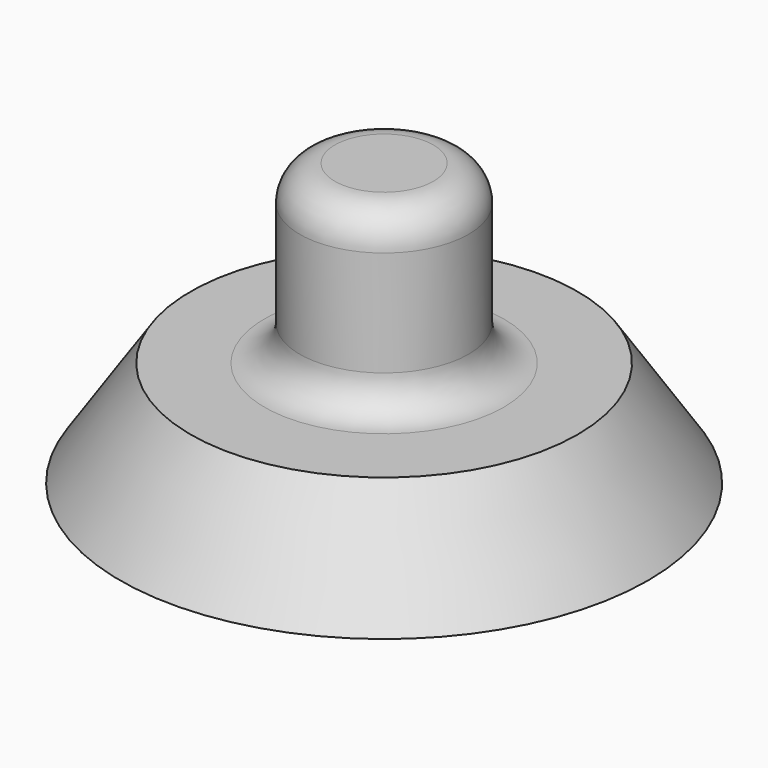
from build123d import *

# Parameters (mm, degrees)
F0_R     = 7.5
F1_DEPTH = 3
F2_SIZE2 = 2.99999
F2_SIZE  = 1.99999
F3_R     = 2.4
F4_DEPTH = 5
F5_R     = 1


# Not quite as in the source:
# - a fillet or chamfer is up to 0.001 mm smaller than in the source, because OpenCascade refuses the exact size


with BuildPart() as f1:
    # F0 (on Top) → F1 (new body)
    with BuildSketch(Plane.XY):
        Circle(F0_R)
    extrude(amount=F1_DEPTH)

    # F2 (size 2 and 3 in the source; OpenCascade refuses exactly that, so slightly less here)
    f2_edges = [f1.edges().sort_by_distance(p)[0] for p in [
        (-7.5, 0, 3),
    ]]
    f2_side = f1.faces().sort_by_distance((0, 0, 3))[0]
    chamfer(f2_edges, length=F2_SIZE, length2=F2_SIZE2, reference=f2_side)

    # F3 (on face) → F4 (join)
    with BuildSketch(Plane.XY.offset(3)):
        Circle(F3_R)
    extrude(amount=F4_DEPTH)

    # F5
    f5_edges = [f1.edges().sort_by_distance(p)[0] for p in [
        (-2.4, 0, 8),
        (-2.4, 0, 3),
    ]]
    fillet(f5_edges, radius=F5_R)

    # F6 (on Right) → F7 (revolve, cut)
    with BuildSketch(Plane.YZ):
        with BuildLine():
            Line((0, 0), (0, 1))
            ThreePointArc((0, 1), (-18.0312229203, -6.4687770797), (-25.5, -24.5))
            Line((-25.5, -24.5), (0, -24.5))
            Line((0, -24.5), (0, 0))
        make_face()
    revolve(axis=Axis((0, 0, -12.25), (0, 0, -1)), mode=Mode.SUBTRACT)


solid = f1.part
